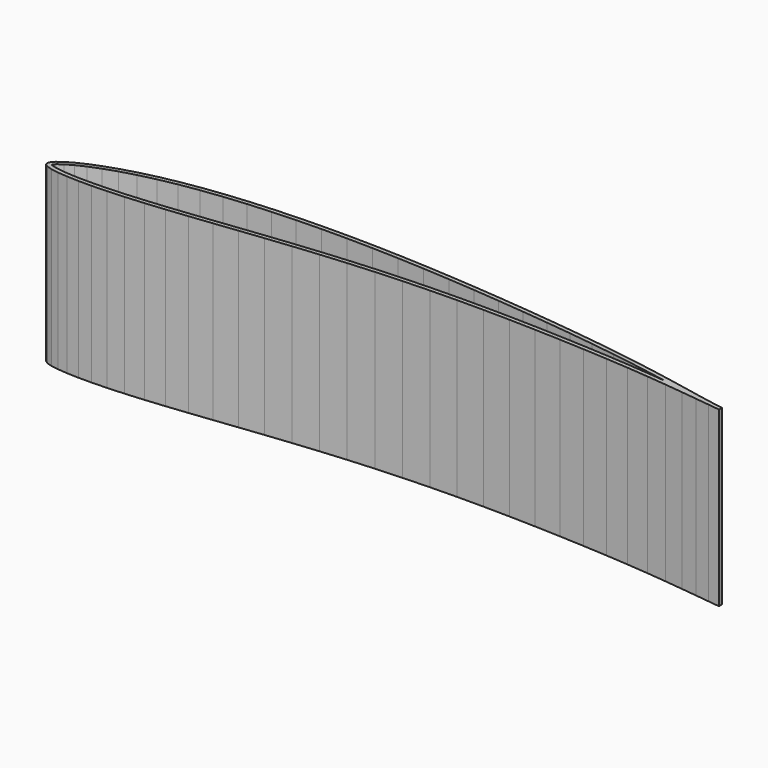
from build123d import *

# Parameters (mm, degrees)
F1_DEPTH = 25
F2_T     = -0.6


# Not quite as in the source:
# - a feature names something its author has since deleted; it is built from what else it names


with BuildPart() as f1:
    # F0 (on Top) → F1 (new body)
    with BuildSketch(Plane.XY):
        Polygon((46.698, -2.739), (46.698, -2.206), (45.044, -1.922), (43.064, -1.555), (40.775, -1.102), (38.202, -0.597), (35.37, -0.07), (35.37, -1.473), (38.202, -1.754), (40.775, -2.038), (43.064, -2.306), (45.044, -2.543), align=None)
        Polygon((35.37, -1.473), (35.37, -0.07), (32.309, 0.453), (29.048, 0.959), (25.616, 1.44), (22.043, 1.892), (18.359, 2.315), (14.594, 2.708), (10.778, 3.069), (6.937, 3.396), (3.099, 3.68), (-0.735, 3.917), (-4.565, 4.101), (-8.362, 4.224), (-12.113, 4.281), (-15.796, 4.268), (-19.391, 4.184), (-22.88, 4.026), (-26.24, 3.795), (-29.451, 3.49), (-32.496, 3.111), (-35.352, 2.66), (-38.001, 2.139), (-40.424, 1.558), (-42.605, 0.932), (-44.532, 0.283), (-46.189, -0.373), (-47.567, -1.019), (-48.662, -1.638), (-49.452, -2.219), (-49.902, -2.749), (-50, -3.09), (-49.902, -3.383), (-49.452, -3.705), (-48.662, -3.939), (-47.567, -4.107), (-46.189, -4.221), (-44.532, -4.281), (-42.605, -4.278), (-40.424, -4.207), (-38.001, -4.067), (-35.352, -3.856), (-32.496, -3.581), (-29.451, -3.25), (-26.24, -2.88), (-22.88, -2.485), (-19.391, -2.083), (-15.796, -1.692), (-12.113, -1.33), (-8.362, -1.011), (-4.565, -0.747), (-0.735, -0.545), (3.099, -0.41), (6.937, -0.339), (10.778, -0.331), (14.594, -0.379), (18.359, -0.477), (22.043, -0.615), (25.616, -0.784), (29.048, -0.983), (32.309, -1.213), align=None)
    extrude(amount=F1_DEPTH)

    # F2
    f2_openings = [f1.faces().sort_by_distance(p)[0] for p in [
        (-12.597329, 0.423659, 25),
    ]]
    offset(amount=F2_T, openings=f2_openings)


solid = f1.part
